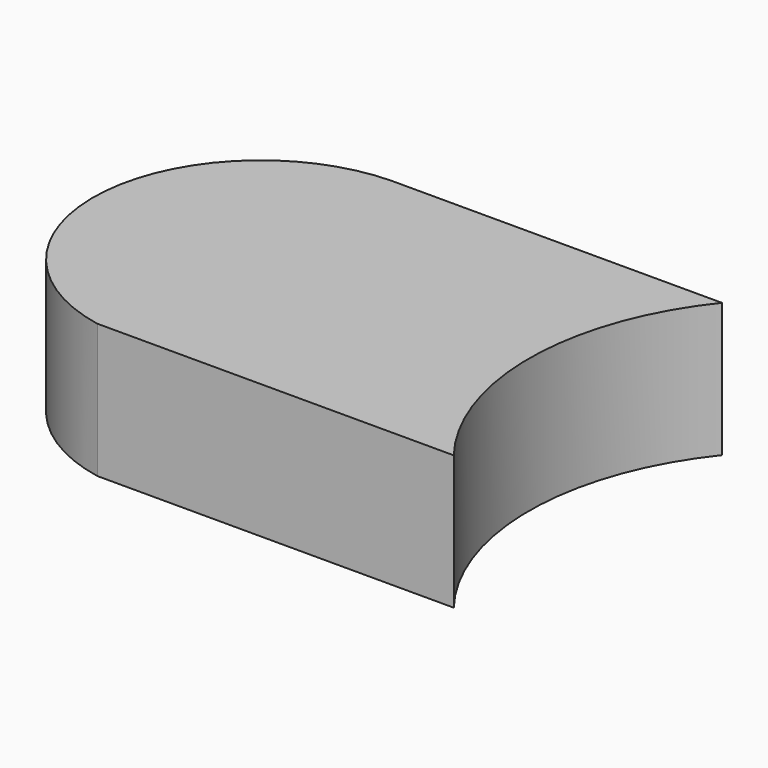
from build123d import *

# Parameters (mm, degrees)
F1_DEPTH = 12.7


# Not quite as in the source:
# - a feature of the source that left no trace in its solid (it failed there, or was rolled back) is left out


with BuildPart() as f1:
    # F0 (on Top) → F1 (new body)
    with BuildSketch(Plane.XY):
        with BuildLine():
            Line((-29.4123420513, 15.8713823409), (-30.0901254618, 15.8713823409))
            ThreePointArc((-30.0901254618, 15.8713823409), (-45.5693436369, 1.3427675948), (-32.7605777455, -15.587157334))
            Line((-32.7605777455, -15.587157334), (-26.7418897676, -15.587157334))
            ThreePointArc((-26.7418897676, -15.587157334), (-17.5080936196, -10.1055007094), (-13.8762337565, 0))
            ThreePointArc((-13.8762337565, 0), (-18.4067300032, 11.1048574772), (-29.4123420513, 15.8713823409))
        make_face()
        with BuildLine():
            Line((1.2180016947, 15.8713823409), (-29.4123420513, 15.8713823409))
            ThreePointArc((-29.4123420513, 15.8713823409), (-18.4067300032, 11.1048574772), (-13.8762337565, 0))
            ThreePointArc((-13.8762337565, 0), (-17.5080936196, -10.1055007094), (-26.7418897676, -15.587157334))
            Line((-26.7418897676, -15.587157334), (0.9938285411, -15.587157334))
            ThreePointArc((0.9938285411, -15.587157334), (-4.350588879, 0.1809954815), (1.2180016947, 15.8713823409))
        make_face()
    extrude(amount=F1_DEPTH)


solid = f1.part
